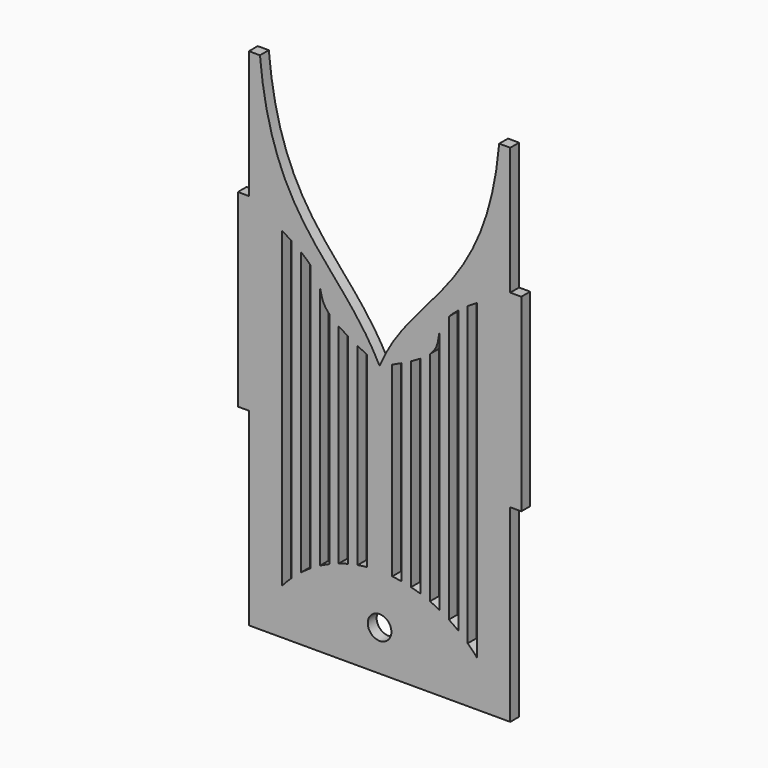
from build123d import *

# Parameters (mm, degrees)
F0_R     = 3.175
F0_W     = 2.9718
F0_H     = 50.8
F0_H_2   = 34.29
F1_DEPTH = 2.9718


# Not quite as in the source:
# - a feature names something its author has since deleted; it is built from what else it names


with BuildPart() as f1:
    # F0 (on Front) → F1 (new body)
    with BuildSketch(Plane.XZ):
        with BuildLine():
            Line((-10.6135604082, -19.6269177035), (-10.6135604082, -70.4269177035))
            Line((-10.6135604082, -70.4269177035), (53.6992395918, -70.4269177035))
            Line((53.6992395918, -70.4269177035), (53.6992395918, -19.6269177035))
            Line((53.6992395918, -19.6269177035), (53.6992395918, 31.1730822965))
            Line((53.6992395918, 31.1730822965), (53.6992395918, 65.4630822965))
            add(Edge.make_bspline(
                [(53.6992395918, 65.4630822965), (50.3210395918, 27.3630822965), (29.9713909626, 22.7711647749), (21.5428395918, 2.3945980662)],
                knots=[0, 0, 0, 0, 70.7931335941, 70.7931335941, 70.7931335941, 70.7931335941], degree=3))
            add(Edge.make_bspline(
                [(-10.6135604082, 65.4630822965), (-7.2353604082, 27.3630822965), (10.8240395918, 23.417426143), (21.5428395918, 2.3945980662)],
                knots=[0, 0, 0, 0, 70.7931335941, 70.7931335941, 70.7931335941, 70.7931335941], degree=3))
            Line((-10.6135604082, 65.4630822965), (-10.6135604082, 31.1730822965))
            Line((-10.6135604082, 31.1730822965), (-10.6135604082, -19.6269177035))
        make_face()
        with Locations((21.5466730297, -59.5008693635)):
            Circle(F0_R, mode=Mode.SUBTRACT)
        with BuildLine():
            add(Edge.make_bspline(
                [(18.174427537, 3.9557799586), (19.2048586468, 3.4597391149), (20.3249139395, 2.9401290525), (21.5428395918, 2.3945980662)],
                knots=[36.4374086053, 36.4374086053, 36.4374086053, 36.4374086053, 38.1, 38.1, 38.1, 38.1], degree=3))
            add(Edge.make_bspline(
                [(24.9210395918, 3.8182866349), (23.8862684635, 3.3648017903), (22.7628335347, 2.8909334778), (21.5428395918, 2.3945980662)],
                knots=[36.4848270835, 36.4848270835, 36.4848270835, 36.4848270835, 38.1, 38.1, 38.1, 38.1], degree=3))
            add(Edge.make_bspline(
                [(27.4610395918, 4.9737252721), (26.6799254221, 4.6035259347), (25.8350725803, 4.2188584101), (24.9210395918, 3.8182866349)],
                knots=[35.0581141735, 35.0581141735, 35.0581141735, 35.0581141735, 36.4848270835, 36.4848270835, 36.4848270835, 36.4848270835], degree=3))
            add(Edge.make_bspline(
                [(30.0010395918, 6.2432045407), (29.2394523696, 5.8391275699), (28.3958951656, 5.4167884341), (27.4610395918, 4.9737252721)],
                knots=[33.3505910381, 33.3505910381, 33.3505910381, 33.3505910381, 35.0581141735, 35.0581141735, 35.0581141735, 35.0581141735], degree=3))
            add(Edge.make_bspline(
                [(32.5410395918, 7.709522157), (31.815508389, 7.2472020661), (30.9753523304, 6.7601477463), (30.0010395918, 6.2432045407)],
                knots=[31.1661248423, 31.1661248423, 31.1661248423, 31.1661248423, 33.3505910381, 33.3505910381, 33.3505910381, 33.3505910381], degree=3))
            add(Edge.make_bspline(
                [(35.0810395918, 9.6243844167), (34.4449246224, 9.0294716961), (33.6196497273, 8.3968297933), (32.5410395918, 7.709522157)],
                knots=[27.9185906625, 27.9185906625, 27.9185906625, 27.9185906625, 31.1661248423, 31.1661248423, 31.1661248423, 31.1661248423], degree=3))
            add(Edge.make_bspline(
                [(37.6210395918, 15.5231181366), (37.1997000639, 13.5029330493), (37.4295721889, 11.8207985618), (35.0810395918, 9.6243844167)],
                knots=[15.9287142288, 15.9287142288, 15.9287142288, 15.9287142288, 27.9185906625, 27.9185906625, 27.9185906625, 27.9185906625], degree=3))
            add(Edge.make_bspline(
                [(40.1610395918, 20.1314996321), (38.4452100282, 18.2956109855), (37.8952324766, 16.8377832468), (37.6210395918, 15.5231181366)],
                knots=[8.1261260785, 8.1261260785, 8.1261260785, 8.1261260785, 15.9287142288, 15.9287142288, 15.9287142288, 15.9287142288], degree=3))
            add(Edge.make_bspline(
                [(42.7010395918, 22.4248035121), (41.6492517803, 21.5958754464), (40.8193404202, 20.8358627241), (40.1610395918, 20.1314996321)],
                knots=[5.1325593794, 5.1325593794, 5.1325593794, 5.1325593794, 8.1261260785, 8.1261260785, 8.1261260785, 8.1261260785], degree=3))
            add(Edge.make_bspline(
                [(45.2410395918, 24.2632398541), (44.2752085711, 23.6139450004), (43.4342172947, 23.0026306826), (42.7010395918, 22.4248035121)],
                knots=[3.0458111478, 3.0458111478, 3.0458111478, 3.0458111478, 5.1325593794, 5.1325593794, 5.1325593794, 5.1325593794], degree=3))
            add(Edge.make_bspline(
                [(47.7810395918, 25.8807627574), (46.8503141861, 25.3162427283), (46.0064724881, 24.7778139666), (45.2410395918, 24.2632398541)],
                knots=[1.3920376526, 1.3920376526, 1.3920376526, 1.3920376526, 3.0458111478, 3.0458111478, 3.0458111478, 3.0458111478], degree=3))
            add(Edge.make_bspline(
                [(50.3210395918, 27.3630822965), (49.4094448692, 26.8496004392), (48.5644629644, 26.3559385528), (47.7810395918, 25.8807627574)],
                knots=[0, 0, 0, 0, 1.3920376526, 1.3920376526, 1.3920376526, 1.3920376526], degree=3))
            Line((50.3210395918, 27.3630822965), (50.3210395918, -61.5369177035))
            ThreePointArc((50.3210395918, -61.5369177035), (49.1018112077, -59.8262756393), (47.7810395918, -58.1927590453))
            ThreePointArc((47.7810395918, -58.1927590453), (46.5462872107, -56.8318592668), (45.2410395918, -55.5384180031))
            ThreePointArc((45.2410395918, -55.5384180031), (43.9971682474, -54.4248535099), (42.7010395918, -53.3725739321))
            ThreePointArc((42.7010395918, -53.3725739321), (41.4510857441, -52.4508932423), (40.1610395918, -51.5862194078))
            ThreePointArc((40.1610395918, -51.5862194078), (38.9066725875, -50.8226179021), (37.6210395918, -50.112919627))
            ThreePointArc((37.6210395918, -50.112919627), (36.36326544, -49.4852618571), (35.0810395918, -48.9092002568))
            ThreePointArc((35.0810395918, -48.9092002568), (33.8205009635, -48.4023559957), (32.5410395918, -47.9453796977))
            ThreePointArc((32.5410395918, -47.9453796977), (31.2781609586, -47.5487876175), (30.0010395918, -47.2007808145))
            ThreePointArc((30.0010395918, -47.2007808145), (28.7361037745, -46.907078004), (27.4610395918, -46.6610387941))
            ThreePointArc((27.4610395918, -46.6610387941), (26.1942303865, -46.4652554761), (24.9210395918, -46.316521248))
            ThreePointArc((24.9210395918, -46.316521248), (21.547756981, -46.1512435423), (18.174427537, -46.3155626059))
            ThreePointArc((18.174427537, -46.3155626059), (16.901243708, -46.46392835), (15.634427537, -46.659341362))
            ThreePointArc((15.634427537, -46.659341362), (14.3593708721, -46.90499798), (13.094427537, -47.1983152681))
            ThreePointArc((13.094427537, -47.1983152681), (11.8173145662, -47.5459173972), (10.554427537, -47.9421006017))
            ThreePointArc((10.554427537, -47.9421006017), (9.2749758876, -48.3986398999), (8.014427537, -48.9050414301))
            ThreePointArc((8.014427537, -48.9050414301), (6.7322134008, -49.480619628), (5.474427537, -50.1077863311))
            ThreePointArc((5.474427537, -50.1077863311), (4.1888093009, -50.8169340928), (2.934427537, -51.5799748434))
            ThreePointArc((2.934427537, -51.5799748434), (1.6444010223, -52.4439982142), (0.394427537, -53.365014544))
            ThreePointArc((0.394427537, -53.365014544), (-0.9016730983, -54.4164866486), (-2.145572463, -55.5292241802))
            ThreePointArc((-2.145572463, -55.5292241802), (-3.4507759715, -56.8215888342), (-4.685572463, -58.1813830179))
            ThreePointArc((-4.685572463, -58.1813830179), (-6.0115928229, -59.8203006816), (-7.2353604082, -61.5369177035))
            add(Edge.make_bspline(
                [(-7.2353604082, 27.3630822965), (-7.2353604082, -0.334873893), (-7.2353604082, -33.838961514), (-7.2353604082, -61.5369177035)],
                knots=[0, 0, 0, 0, 88.9, 88.9, 88.9, 88.9], degree=3))
            add(Edge.make_bspline(
                [(-7.2353604082, 27.3630822965), (-6.3195404997, 26.8524970598), (-5.4713701457, 26.3626827218), (-4.685572463, 25.8921343821)],
                knots=[0, 0, 0, 0, 1.4327172124, 1.4327172124, 1.4327172124, 1.4327172124], degree=3))
            add(Edge.make_bspline(
                [(-4.685572463, 25.8921343821), (-3.7542137819, 25.3344217663), (-2.9104758153, 24.8037738972), (-2.145572463, 24.29768509)],
                knots=[1.4327172124, 1.4327172124, 1.4327172124, 1.4327172124, 3.1308306617, 3.1308306617, 3.1308306617, 3.1308306617], degree=3))
            add(Edge.make_bspline(
                [(-2.145572463, 24.29768509), (-1.1789086721, 23.6581039933), (-0.3381532858, 23.057746686), (0.394427537, 22.491555701)],
                knots=[3.1308306617, 3.1308306617, 3.1308306617, 3.1308306617, 5.2768596724, 5.2768596724, 5.2768596724, 5.2768596724], degree=3))
            add(Edge.make_bspline(
                [(0.394427537, 22.491555701), (1.4468013348, 21.6782057761), (2.2759443341, 20.9353620327), (2.934427537, 20.2480318861)],
                knots=[5.2768596724, 5.2768596724, 5.2768596724, 5.2768596724, 8.3596931702, 8.3596931702, 8.3596931702, 8.3596931702], degree=3))
            add(Edge.make_bspline(
                [(2.934427537, 20.2480318861), (4.5480124747, 18.5637587463), (5.1368295827, 17.2128303622), (5.474427537, 15.9746404386)],
                knots=[8.3596931702, 8.3596931702, 8.3596931702, 8.3596931702, 15.9140448616, 15.9140448616, 15.9140448616, 15.9140448616], degree=3))
            add(Edge.make_bspline(
                [(5.474427537, 15.9746404386), (5.9896552573, 14.084967342), (5.9197540389, 12.4578798594), (8.014427537, 10.3091972977)],
                knots=[15.9140448616, 15.9140448616, 15.9140448616, 15.9140448616, 27.4431769284, 27.4431769284, 27.4431769284, 27.4431769284], degree=3))
            add(Edge.make_bspline(
                [(8.014427537, 10.3091972977), (8.6420846531, 9.6653566698), (9.4640918921, 8.9746837165), (10.554427537, 8.2160807673)],
                knots=[27.4431769284, 27.4431769284, 27.4431769284, 27.4431769284, 30.8978164182, 30.8978164182, 30.8978164182, 30.8978164182], degree=3))
            add(Edge.make_bspline(
                [(10.554427537, 8.2160807673), (11.2763160606, 7.713825553), (12.1158260279, 7.1817933043), (13.094427537, 6.6138610208)],
                knots=[30.8978164182, 30.8978164182, 30.8978164182, 30.8978164182, 33.1850612795, 33.1850612795, 33.1850612795, 33.1850612795], degree=3))
            add(Edge.make_bspline(
                [(13.094427537, 6.6138610208), (13.8539601424, 6.1730655764), (14.6972807439, 5.7106441444), (15.634427537, 5.2237339583)],
                knots=[33.1850612795, 33.1850612795, 33.1850612795, 33.1850612795, 34.9602854465, 34.9602854465, 34.9602854465, 34.9602854465], degree=3))
            add(Edge.make_bspline(
                [(15.634427537, 5.2237339583), (16.4142058077, 4.8185872026), (17.2589448389, 4.3964856066), (18.174427537, 3.9557799586)],
                knots=[34.9602854465, 34.9602854465, 34.9602854465, 34.9602854465, 36.4374086053, 36.4374086053, 36.4374086053, 36.4374086053], degree=3))
        make_face(mode=Mode.SUBTRACT)
        with BuildLine():
            add(Edge.make_bspline(
                [(24.9210395918, 3.8182866349), (23.8862684635, 3.3648017903), (22.7628335347, 2.8909334778), (21.5428395918, 2.3945980662)],
                knots=[36.4848270835, 36.4848270835, 36.4848270835, 36.4848270835, 38.1, 38.1, 38.1, 38.1], degree=3))
            add(Edge.make_bspline(
                [(18.174427537, 3.9557799586), (19.2048586468, 3.4597391149), (20.3249139395, 2.9401290525), (21.5428395918, 2.3945980662)],
                knots=[36.4374086053, 36.4374086053, 36.4374086053, 36.4374086053, 38.1, 38.1, 38.1, 38.1], degree=3))
            Line((18.174427537, 3.9557799586), (18.174427537, -46.3155626059))
            ThreePointArc((18.174427537, -46.3155626059), (21.547756981, -46.1512435423), (24.9210395918, -46.316521248))
            Line((24.9210395918, -46.316521248), (24.9210395918, 3.8182866349))
        make_face()
        with BuildLine():
            Line((-4.685572463, -58.1813830179), (-4.685572463, 25.8921343821))
            add(Edge.make_bspline(
                [(-7.2353604082, 27.3630822965), (-6.3195404997, 26.8524970598), (-5.4713701457, 26.3626827218), (-4.685572463, 25.8921343821)],
                knots=[0, 0, 0, 0, 1.4327172124, 1.4327172124, 1.4327172124, 1.4327172124], degree=3))
            add(Edge.make_bspline(
                [(-7.2353604082, 27.3630822965), (-7.2353604082, -0.334873893), (-7.2353604082, -33.838961514), (-7.2353604082, -61.5369177035)],
                knots=[0, 0, 0, 0, 88.9, 88.9, 88.9, 88.9], degree=3))
            ThreePointArc((-7.2353604082, -61.5369177035), (-6.0115928229, -59.8203006816), (-4.685572463, -58.1813830179))
        make_face()
        with BuildLine():
            add(Edge.make_bspline(
                [(50.3210395918, 27.3630822965), (49.4094448692, 26.8496004392), (48.5644629644, 26.3559385528), (47.7810395918, 25.8807627574)],
                knots=[0, 0, 0, 0, 1.3920376526, 1.3920376526, 1.3920376526, 1.3920376526], degree=3))
            Line((47.7810395918, 25.8807627574), (47.7810395918, -58.1927590453))
            ThreePointArc((47.7810395918, -58.1927590453), (49.1018112077, -59.8262756393), (50.3210395918, -61.5369177035))
            Line((50.3210395918, -61.5369177035), (50.3210395918, 27.3630822965))
        make_face()
        with BuildLine():
            Line((0.394427537, -53.365014544), (0.394427537, 22.491555701))
            add(Edge.make_bspline(
                [(-2.145572463, 24.29768509), (-1.1789086721, 23.6581039933), (-0.3381532858, 23.057746686), (0.394427537, 22.491555701)],
                knots=[3.1308306617, 3.1308306617, 3.1308306617, 3.1308306617, 5.2768596724, 5.2768596724, 5.2768596724, 5.2768596724], degree=3))
            Line((-2.145572463, 24.29768509), (-2.145572463, -55.5292241802))
            ThreePointArc((-2.145572463, -55.5292241802), (-0.9016730983, -54.4164866486), (0.394427537, -53.365014544))
        make_face()
        with BuildLine():
            add(Edge.make_bspline(
                [(45.2410395918, 24.2632398541), (44.2752085711, 23.6139450004), (43.4342172947, 23.0026306826), (42.7010395918, 22.4248035121)],
                knots=[3.0458111478, 3.0458111478, 3.0458111478, 3.0458111478, 5.1325593794, 5.1325593794, 5.1325593794, 5.1325593794], degree=3))
            Line((42.7010395918, 22.4248035121), (42.7010395918, -53.3725739321))
            ThreePointArc((42.7010395918, -53.3725739321), (43.9971682474, -54.4248535099), (45.2410395918, -55.5384180031))
            Line((45.2410395918, -55.5384180031), (45.2410395918, 24.2632398541))
        make_face()
        with BuildLine():
            Line((5.474427537, -50.1077863311), (5.474427537, 15.9746404386))
            add(Edge.make_bspline(
                [(2.934427537, 20.2480318861), (4.5480124747, 18.5637587463), (5.1368295827, 17.2128303622), (5.474427537, 15.9746404386)],
                knots=[8.3596931702, 8.3596931702, 8.3596931702, 8.3596931702, 15.9140448616, 15.9140448616, 15.9140448616, 15.9140448616], degree=3))
            Line((2.934427537, 20.2480318861), (2.934427537, -51.5799748434))
            ThreePointArc((2.934427537, -51.5799748434), (4.1888093009, -50.8169340928), (5.474427537, -50.1077863311))
        make_face()
        with BuildLine():
            add(Edge.make_bspline(
                [(40.1610395918, 20.1314996321), (38.4452100282, 18.2956109855), (37.8952324766, 16.8377832468), (37.6210395918, 15.5231181366)],
                knots=[8.1261260785, 8.1261260785, 8.1261260785, 8.1261260785, 15.9287142288, 15.9287142288, 15.9287142288, 15.9287142288], degree=3))
            Line((37.6210395918, 15.5231181366), (37.6210395918, -50.112919627))
            ThreePointArc((37.6210395918, -50.112919627), (38.9066725875, -50.8226179021), (40.1610395918, -51.5862194078))
            Line((40.1610395918, -51.5862194078), (40.1610395918, 20.1314996321))
        make_face()
        with Locations((55.1851395918, 5.7730822965)):
            Rectangle(F0_W, F0_H)
        with Locations((-12.0994604082, 5.7730822965)):
            Rectangle(F0_W, F0_H)
        with Locations((-15.0712604082, 5.7730822965)):
            Rectangle(F0_W, F0_H)
        with Locations((-12.0994604082, -45.0269177035)):
            Rectangle(F0_W, F0_H)
        with Locations((55.1851395918, -45.0269177035)):
            Rectangle(F0_W, F0_H)
        with Locations((58.1569395918, 5.7730822965)):
            Rectangle(F0_W, F0_H)
        with BuildLine():
            Line((10.554427537, -47.9421006017), (10.554427537, 8.2160807673))
            add(Edge.make_bspline(
                [(8.014427537, 10.3091972977), (8.6420846531, 9.6653566698), (9.4640918921, 8.9746837165), (10.554427537, 8.2160807673)],
                knots=[27.4431769284, 27.4431769284, 27.4431769284, 27.4431769284, 30.8978164182, 30.8978164182, 30.8978164182, 30.8978164182], degree=3))
            Line((8.014427537, 10.3091972977), (8.014427537, -48.9050414301))
            ThreePointArc((8.014427537, -48.9050414301), (9.2749758876, -48.3986398999), (10.554427537, -47.9421006017))
        make_face()
        with BuildLine():
            add(Edge.make_bspline(
                [(35.0810395918, 9.6243844167), (34.4449246224, 9.0294716961), (33.6196497273, 8.3968297933), (32.5410395918, 7.709522157)],
                knots=[27.9185906625, 27.9185906625, 27.9185906625, 27.9185906625, 31.1661248423, 31.1661248423, 31.1661248423, 31.1661248423], degree=3))
            Line((32.5410395918, 7.709522157), (32.5410395918, -47.9453796977))
            ThreePointArc((32.5410395918, -47.9453796977), (33.8205009635, -48.4023559957), (35.0810395918, -48.9092002568))
            Line((35.0810395918, -48.9092002568), (35.0810395918, 9.6243844167))
        make_face()
        with BuildLine():
            Line((15.634427537, -46.659341362), (15.634427537, 5.2237339583))
            add(Edge.make_bspline(
                [(13.094427537, 6.6138610208), (13.8539601424, 6.1730655764), (14.6972807439, 5.7106441444), (15.634427537, 5.2237339583)],
                knots=[33.1850612795, 33.1850612795, 33.1850612795, 33.1850612795, 34.9602854465, 34.9602854465, 34.9602854465, 34.9602854465], degree=3))
            Line((13.094427537, 6.6138610208), (13.094427537, -47.1983152681))
            ThreePointArc((13.094427537, -47.1983152681), (14.3593708721, -46.90499798), (15.634427537, -46.659341362))
        make_face()
        with BuildLine():
            add(Edge.make_bspline(
                [(30.0010395918, 6.2432045407), (29.2394523696, 5.8391275699), (28.3958951656, 5.4167884341), (27.4610395918, 4.9737252721)],
                knots=[33.3505910381, 33.3505910381, 33.3505910381, 33.3505910381, 35.0581141735, 35.0581141735, 35.0581141735, 35.0581141735], degree=3))
            Line((27.4610395918, 4.9737252721), (27.4610395918, -46.6610387941))
            ThreePointArc((27.4610395918, -46.6610387941), (28.7361037745, -46.907078004), (30.0010395918, -47.2007808145))
            Line((30.0010395918, -47.2007808145), (30.0010395918, 6.2432045407))
        make_face()
        with Locations((-12.0994604082, 48.3180822965)):
            Rectangle(F0_W, F0_H_2)
        with Locations((55.1851395918, 48.3180822965)):
            Rectangle(F0_W, F0_H_2)
    extrude(amount=F1_DEPTH)


solid = f1.part
